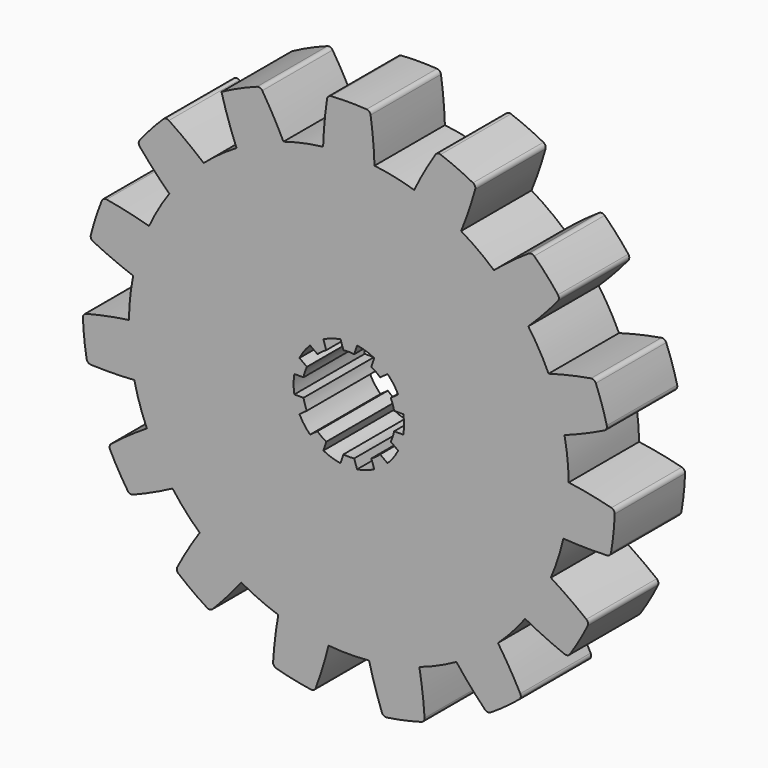
from build123d import *

# Parameters (mm, degrees)
F0_R     = 50
F1_DEPTH = 20
F2_DEPTH = 20
F4_DEPTH = 20
F5_R     = 1


with BuildPart() as f1:
    # F0 (on Front) → F1 (new body)
    with BuildSketch(Plane.XZ):
        Circle(F0_R)
        with BuildLine():
            ThreePointArc((12.3814377194, 2.05), (12.5077884412, 1.0284591925), (12.55, 0))
            ThreePointArc((12.55, 0), (12.5077884412, -1.0284591925), (12.3814377194, -2.05))
            ThreePointArc((12.3814377194, -2.05), (11.9357592795, -3.8781632794), (11.221753297, -5.6191416552))
            ThreePointArc((11.221753297, -5.6191416552), (10.1531632794, -7.3767049163), (8.8118337626, -8.9361113321))
            ThreePointArc((8.8118337626, -8.9361113321), (7.3767049163, -10.1531632794), (5.7757405285, -11.1419621857))
            ThreePointArc((5.7757405285, -11.1419621857), (3.8781632794, -11.9357592795), (1.8764088117, -12.4089318626))
            ThreePointArc((1.8764088117, -12.4089318626), (0, -12.55), (-1.8764088117, -12.4089318626))
            ThreePointArc((-1.8764088117, -12.4089318626), (-3.8781632794, -11.9357592795), (-5.7757405285, -11.1419621857))
            ThreePointArc((-5.7757405285, -11.1419621857), (-7.3767049163, -10.1531632794), (-8.8118337626, -8.9361113321))
            ThreePointArc((-8.8118337626, -8.9361113321), (-10.1531632794, -7.3767049163), (-11.221753297, -5.6191416552))
            ThreePointArc((-11.221753297, -5.6191416552), (-11.9357592795, -3.8781632794), (-12.3814377194, -2.05))
            ThreePointArc((-12.3814377194, -2.05), (-12.55, 0), (-12.3814377194, 2.05))
            ThreePointArc((-12.3814377194, 2.05), (-11.9357592795, 3.8781632794), (-11.221753297, 5.6191416552))
            ThreePointArc((-11.221753297, 5.6191416552), (-10.1531632794, 7.3767049163), (-8.8118337626, 8.9361113321))
            ThreePointArc((-8.8118337626, 8.9361113321), (-7.3767049163, 10.1531632794), (-5.7757405285, 11.1419621857))
            ThreePointArc((-5.7757405285, 11.1419621857), (-3.8781632794, 11.9357592795), (-1.8764088117, 12.4089318626))
            ThreePointArc((-1.8764088117, 12.4089318626), (0, 12.55), (1.8764088117, 12.4089318626))
            ThreePointArc((1.8764088117, 12.4089318626), (3.8781632794, 11.9357592795), (5.7757405285, 11.1419621857))
            ThreePointArc((5.7757405285, 11.1419621857), (7.3767049163, 10.1531632794), (8.8118337626, 8.9361113321))
            ThreePointArc((8.8118337626, 8.9361113321), (10.1531632794, 7.3767049163), (11.221753297, 5.6191416552))
            ThreePointArc((11.221753297, 5.6191416552), (11.9357592795, 3.8781632794), (12.3814377194, 2.05))
        make_face(mode=Mode.SUBTRACT)
    extrude(amount=F1_DEPTH)

    # F0 (on Front) → F2 (join)
    with BuildSketch(Plane.XZ):
        with BuildLine():
            Line((10.2979366865, 2.05), (12.3814377194, 2.05))
            ThreePointArc((12.3814377194, 2.05), (11.9357592795, 3.8781632794), (11.221753297, 5.6191416552))
            Line((11.221753297, 5.6191416552), (9.5361655536, 4.3944904749))
            ThreePointArc((9.5361655536, 4.3944904749), (9.9860934211, 3.2446784409), (10.2979366865, 2.05))
        make_face()
        with BuildLine():
            ThreePointArc((11.221753297, -5.6191416552), (11.9357592795, -3.8781632794), (12.3814377194, -2.05))
            Line((12.3814377194, -2.05), (10.2979366865, -2.05))
            ThreePointArc((10.2979366865, -2.05), (9.9860934211, -3.2446784409), (9.5361655536, -4.3944904749))
            Line((9.5361655536, -4.3944904749), (11.221753297, -5.6191416552))
        make_face()
        with BuildLine():
            Line((7.1262460192, 7.7114601519), (8.8118337626, 8.9361113321))
            ThreePointArc((8.8118337626, 8.9361113321), (7.3767049163, 10.1531632794), (5.7757405285, 11.1419621857))
            Line((5.7757405285, 11.1419621857), (5.1319033015, 9.1604349517))
            ThreePointArc((5.1319033015, 9.1604349517), (6.1717451491, 8.4946784409), (7.1262460192, 7.7114601519))
        make_face()
        with BuildLine():
            ThreePointArc((5.7757405285, -11.1419621857), (7.3767049163, -10.1531632794), (8.8118337626, -8.9361113321))
            Line((8.8118337626, -8.9361113321), (7.1262460192, -7.7114601519))
            ThreePointArc((7.1262460192, -7.7114601519), (6.1717451491, -8.4946784409), (5.1319033015, -9.1604349517))
            Line((5.1319033015, -9.1604349517), (5.7757405285, -11.1419621857))
        make_face()
        with BuildLine():
            Line((1.2325715847, 10.4274046286), (1.8764088117, 12.4089318626))
            ThreePointArc((1.8764088117, 12.4089318626), (0, 12.55), (-1.8764088117, 12.4089318626))
            Line((-1.8764088117, 12.4089318626), (-1.2325715847, 10.4274046286))
            ThreePointArc((-1.2325715847, 10.4274046286), (0, 10.5), (1.2325715847, 10.4274046286))
        make_face()
        with BuildLine():
            ThreePointArc((-1.8764088117, -12.4089318626), (0, -12.55), (1.8764088117, -12.4089318626))
            Line((1.8764088117, -12.4089318626), (1.2325715847, -10.4274046286))
            ThreePointArc((1.2325715847, -10.4274046286), (0, -10.5), (-1.2325715847, -10.4274046286))
            Line((-1.2325715847, -10.4274046286), (-1.8764088117, -12.4089318626))
        make_face()
        with BuildLine():
            Line((-5.1319033015, 9.1604349517), (-5.7757405285, 11.1419621857))
            ThreePointArc((-5.7757405285, 11.1419621857), (-7.3767049163, 10.1531632794), (-8.8118337626, 8.9361113321))
            Line((-8.8118337626, 8.9361113321), (-7.1262460192, 7.7114601519))
            ThreePointArc((-7.1262460192, 7.7114601519), (-6.1717451491, 8.4946784409), (-5.1319033015, 9.1604349517))
        make_face()
        with BuildLine():
            ThreePointArc((-8.8118337626, -8.9361113321), (-7.3767049163, -10.1531632794), (-5.7757405285, -11.1419621857))
            Line((-5.7757405285, -11.1419621857), (-5.1319033015, -9.1604349517))
            ThreePointArc((-5.1319033015, -9.1604349517), (-6.1717451491, -8.4946784409), (-7.1262460192, -7.7114601519))
            Line((-7.1262460192, -7.7114601519), (-8.8118337626, -8.9361113321))
        make_face()
        with BuildLine():
            Line((-9.5361655536, 4.3944904749), (-11.221753297, 5.6191416552))
            ThreePointArc((-11.221753297, 5.6191416552), (-11.9357592795, 3.8781632794), (-12.3814377194, 2.05))
            Line((-12.3814377194, 2.05), (-10.2979366865, 2.05))
            ThreePointArc((-10.2979366865, 2.05), (-9.9860934211, 3.2446784409), (-9.5361655536, 4.3944904749))
        make_face()
        with BuildLine():
            ThreePointArc((-12.3814377194, -2.05), (-11.9357592795, -3.8781632794), (-11.221753297, -5.6191416552))
            Line((-11.221753297, -5.6191416552), (-9.5361655536, -4.3944904749))
            ThreePointArc((-9.5361655536, -4.3944904749), (-9.9860934211, -3.2446784409), (-10.2979366865, -2.05))
            Line((-10.2979366865, -2.05), (-12.3814377194, -2.05))
        make_face()
    extrude(amount=F2_DEPTH)

    # F3 (on Front) → F4 (join)
    with BuildSketch(Plane.XZ):
        with BuildLine():
            ThreePointArc((-5.844604574, 49.6572310683), (0, 50), (5.844604574, 49.6572310683))
            ThreePointArc((5.844604574, 49.6572310683), (5.4980069733, 54.9968903966), (4.8346959965, 60.3065146947))
            ThreePointArc((4.8346959965, 60.3065146947), (0, 60.5), (-4.8346959965, 60.3065146947))
            ThreePointArc((-4.8346959965, 60.3065146947), (-5.4980069733, 54.9968903966), (-5.844604574, 49.6572310683))
        make_face()
        with BuildLine():
            ThreePointArc((14.8581035088, 47.7413527261), (20.3368321538, 45.6772728821), (25.5367274295, 42.986923037))
            ThreePointArc((25.5367274295, 42.986923037), (27.3919298761, 48.0059185064), (28.9455839092, 53.1262945457))
            ThreePointArc((28.9455839092, 53.1262945457), (24.6075669061, 55.2695001874), (20.1121547759, 57.0591905855))
            ThreePointArc((20.1121547759, 57.0591905855), (17.346571283, 52.4784003062), (14.8581035088, 47.7413527261))
        make_face()
        with BuildLine():
            ThreePointArc((32.9917105134, 37.570560781), (37.1572412739, 33.4565303179), (40.8133181185, 28.8837854887))
            ThreePointArc((40.8133181185, 28.8837854887), (44.5495392554, 32.7142871863), (48.0515174016, 36.7600554325))
            ThreePointArc((48.0515174016, 36.7600554325), (44.9602619414, 40.4824016847), (41.5814312743, 43.9458140576))
            ThreePointArc((41.5814312743, 43.9458140576), (37.1917697758, 40.8859180516), (32.9917105134, 37.570560781))
        make_face()
        with BuildLine():
            ThreePointArc((45.4207510499, 20.903477559), (47.5528258148, 15.4508497187), (49.0329153275, 9.7863790284))
            ThreePointArc((49.0329153275, 9.7863790284), (54.0041285776, 11.7660584117), (58.848907001, 14.0376687804))
            ThreePointArc((58.848907001, 14.0376687804), (57.5389192359, 18.6955281597), (55.8609005499, 23.2338070439))
            ThreePointArc((55.8609005499, 23.2338070439), (50.6061733977, 22.2238891289), (45.4207510499, 20.903477559))
        make_face()
        with BuildLine():
            ThreePointArc((49.9961310953, 0.621993165), (49.9990327645, 0.3110025987), (50, 0))
            ThreePointArc((50, 0), (49.6926242078, -5.5356209537), (48.7742760263, -11.0031812724))
            ThreePointArc((48.7742760263, -11.0031812724), (54.1209134566, -11.2166287535), (59.4707859543, -11.111958332))
            ThreePointArc((59.4707859543, -11.111958332), (60.1685746698, -6.3239720277), (60.4815126401, -1.4955362801))
            ThreePointArc((60.4815126401, -1.4955362801), (55.2703098965, -0.2808521218), (49.9961310953, 0.621993165))
        make_face()
        with BuildLine():
            ThreePointArc((54.6443217375, -25.9662877948), (50.3777076993, -22.7370314892), (45.9267258738, -19.767039498))
            ThreePointArc((45.9267258738, -19.767039498), (43.3012701892, -25), (40.0821212997, -29.8901915704))
            ThreePointArc((40.0821212997, -29.8901915704), (44.879700726, -32.2598589074), (49.8096257411, -34.3402268999))
            ThreePointArc((49.8096257411, -34.3402268999), (52.394536929, -30.25), (54.6443217375, -25.9662877948))
        make_face()
        with BuildLine():
            ThreePointArc((39.3586311785, -45.9472322535), (36.7743421737, -41.2617715527), (33.9161725174, -36.7381714538))
            ThreePointArc((33.9161725174, -36.7381714538), (29.3892626146, -40.4508497187), (24.4594036658, -43.608916202))
            ThreePointArc((24.4594036658, -43.608916202), (27.8783800205, -47.7250663845), (31.5359287309, -51.6307582656))
            ThreePointArc((31.5359287309, -51.6307582656), (35.5610077637, -48.9455281597), (39.3586311785, -45.9472322535))
        make_face()
        with BuildLine():
            ThreePointArc((17.2674757267, -57.983482838), (16.8123588018, -52.6519764633), (16.0412048141, -47.3569398094))
            ThreePointArc((16.0412048141, -47.3569398094), (10.3955845409, -48.9073800367), (4.6074329314, -49.7872630477))
            ThreePointArc((4.6074329314, -49.7872630477), (6.0566341423, -54.9381763152), (7.8093831483, -59.9938624765))
            ThreePointArc((7.8093831483, -59.9938624765), (12.5786572945, -59.1779298444), (17.2674757267, -57.983482838))
        make_face()
        with BuildLine():
            ThreePointArc((-7.8093831483, -59.9938624765), (-6.0566341423, -54.9381763152), (-4.6074329314, -49.7872630477))
            ThreePointArc((-4.6074329314, -49.7872630477), (-10.3955845409, -48.9073800367), (-16.0412048141, -47.3569398094))
            ThreePointArc((-16.0412048141, -47.3569398094), (-16.8123588018, -52.6519764633), (-17.2674757267, -57.983482838))
            ThreePointArc((-17.2674757267, -57.983482838), (-12.5786572945, -59.1779298444), (-7.8093831483, -59.9938624765))
        make_face()
        with BuildLine():
            ThreePointArc((-31.5359287309, -51.6307582656), (-27.8783800205, -47.7250663845), (-24.4594036658, -43.608916202))
            ThreePointArc((-24.4594036658, -43.608916202), (-29.3892626146, -40.4508497187), (-33.9161725174, -36.7381714538))
            ThreePointArc((-33.9161725174, -36.7381714538), (-36.7743421737, -41.2617715527), (-39.3586311785, -45.9472322535))
            ThreePointArc((-39.3586311785, -45.9472322535), (-35.5610077637, -48.9455281597), (-31.5359287309, -51.6307582656))
        make_face()
        with BuildLine():
            ThreePointArc((-49.8096257411, -34.3402268999), (-44.879700726, -32.2598589074), (-40.0821212997, -29.8901915704))
            ThreePointArc((-40.0821212997, -29.8901915704), (-43.3012701892, -25), (-45.9267258738, -19.767039498))
            ThreePointArc((-45.9267258738, -19.767039498), (-50.3777076993, -22.7370314892), (-54.6443217375, -25.9662877948))
            ThreePointArc((-54.6443217375, -25.9662877948), (-52.394536929, -30.25), (-49.8096257411, -34.3402268999))
        make_face()
        with BuildLine():
            ThreePointArc((-59.4707859543, -11.111958332), (-54.1209134566, -11.2166287535), (-48.7742760263, -11.0031812724))
            ThreePointArc((-48.7742760263, -11.0031812724), (-49.7260947684, -5.2264231634), (-49.9961310953, 0.621993165))
            ThreePointArc((-49.9961310953, 0.621993165), (-55.2703098965, -0.2808521218), (-60.4815126401, -1.4955362801))
            ThreePointArc((-60.4815126401, -1.4955362801), (-60.1685746698, -6.3239720277), (-59.4707859543, -11.111958332))
        make_face()
        with BuildLine():
            ThreePointArc((-25.5367274295, 42.986923037), (-20.3368321538, 45.6772728821), (-14.8581035088, 47.7413527261))
            ThreePointArc((-14.8581035088, 47.7413527261), (-17.346571283, 52.4784003062), (-20.1121547759, 57.0591905855))
            ThreePointArc((-20.1121547759, 57.0591905855), (-24.6075669061, 55.2695001874), (-28.9455839092, 53.1262945457))
            ThreePointArc((-28.9455839092, 53.1262945457), (-27.3919298761, 48.0059185064), (-25.5367274295, 42.986923037))
        make_face()
        with BuildLine():
            ThreePointArc((-40.8133181185, 28.8837854887), (-37.1572412739, 33.4565303179), (-32.9917105134, 37.570560781))
            ThreePointArc((-32.9917105134, 37.570560781), (-37.1917697758, 40.8859180516), (-41.5814312743, 43.9458140576))
            ThreePointArc((-41.5814312743, 43.9458140576), (-44.9602619414, 40.4824016847), (-48.0515174016, 36.7600554325))
            ThreePointArc((-48.0515174016, 36.7600554325), (-44.5495392554, 32.7142871863), (-40.8133181185, 28.8837854887))
        make_face()
        with BuildLine():
            ThreePointArc((-49.0329153275, 9.7863790284), (-47.5528258148, 15.4508497187), (-45.4207510499, 20.903477559))
            ThreePointArc((-45.4207510499, 20.903477559), (-50.6061733977, 22.2238891289), (-55.8609005499, 23.2338070439))
            ThreePointArc((-55.8609005499, 23.2338070439), (-57.5389192359, 18.6955281597), (-58.848907001, 14.0376687804))
            ThreePointArc((-58.848907001, 14.0376687804), (-54.0041285776, 11.7660584117), (-49.0329153275, 9.7863790284))
        make_face()
    extrude(amount=F4_DEPTH)

    # F5
    f5_edges = [f1.edges().sort_by_distance(p)[0] for p in [
        (-31.535929, -10, -51.630758),
        (-17.267476, -10, -57.983483),
        (-7.809383, -10, -59.993862),
        (7.809383, -10, -59.993862),
        (17.267476, -10, -57.983483),
        (31.535929, -10, -51.630758),
        (39.358631, -10, -45.947232),
        (49.809626, -10, -34.340227),
        (54.644322, -10, -25.966288),
        (59.470786, -10, -11.111958),
        (60.481513, -10, -1.495536),
        (58.848907, -10, 14.037669),
        (55.860901, -10, 23.233807),
        (48.051517, -10, 36.760055),
        (41.581431, -10, 43.945814),
        (28.945584, -10, 53.126295),
        (20.112155, -10, 57.059191),
        (4.834696, -10, 60.306515),
        (-4.834696, -10, 60.306515),
        (-20.112155, -10, 57.059191),
        (-41.581431, -10, 43.945814),
        (-48.051517, -10, 36.760055),
        (-55.860901, -10, 23.233807),
        (-58.848907, -10, 14.037669),
        (-60.481513, -10, -1.495536),
        (-59.470786, -10, -11.111958),
        (-54.644322, -10, -25.966288),
        (-49.809626, -10, -34.340227),
        (-39.358631, -10, -45.947232),
    ]]
    fillet(f5_edges, radius=F5_R)


solid = f1.part
